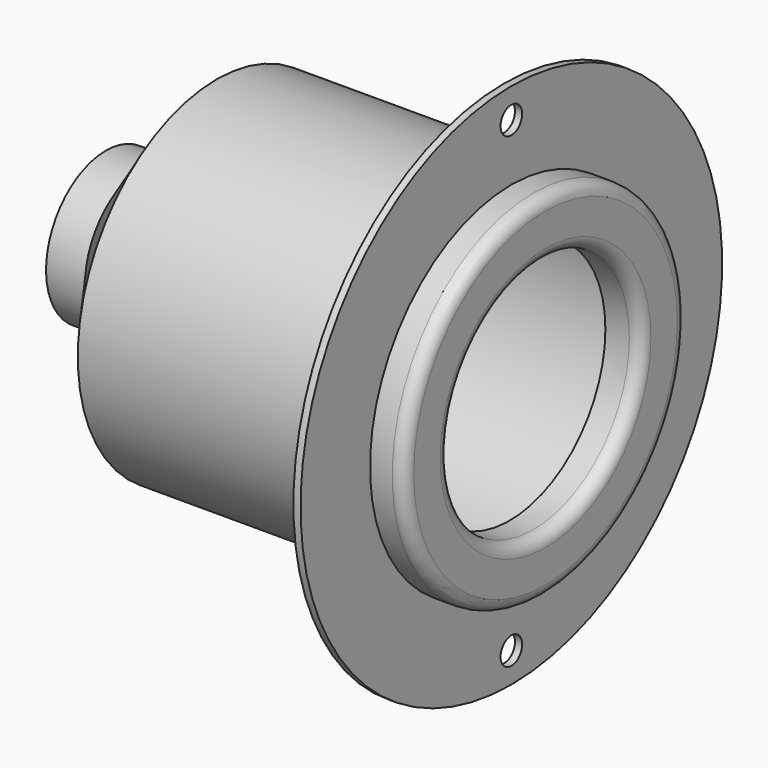
from build123d import *

# Parameters (mm, degrees)
F2_R     = 20
F3_DEPTH = 6
F4_T     = 1
F5_R     = 2
F7_D     = 4.5


# Not quite as in the source:
# - a shell that OpenCascade refuses in one call is made with other operations: the cavity is built on its own and cut out


with BuildPart() as f1:
    # F0 (on Front) → F1 (revolve)
    with BuildSketch(Plane.XZ):
        Polygon((0, 12.5), (0, 0), (73.4, 0), (73.4, 29.5), (67.7, 29.5), (67.7, 44), (66.5, 44), (66.5, 29), (18.5, 29), (6.5, 12.5), align=None)
    revolve(axis=Axis((36.7, 0, 0), (-1, 0, 0)))

    # F2 (on face) → F3 (cut)
    with BuildSketch(Plane.YZ.offset(73.4)):
        Circle(F2_R)
    extrude(amount=-F3_DEPTH, mode=Mode.SUBTRACT)

    # F4: shell of thickness 1, made by hand


with BuildPart() as f4_core1:
    # F4_t2: copy of F1
    add(f1.part)

    # the walls: a layer under each face that stays
    f4_faces = [f4_core1.faces().sort_by_distance(p)[0] for p in [
        (3.25, 0, -12.5),
        (12.5, 0, -20.75),
        (42.5, 0, -29),
        (66.5, -29.3333333333, -29.3333333333),
        (67.1, 0, -44),
        (67.7, -29.3333333333, 29.3333333333),
        (70.55, 0, -29.5),
        (73.4, -19.6666666667, 19.6666666667),
        (70.4, -20, 0),
    ]]
    thicken(f4_faces, amount=-F4_T, mode=Mode.SUBTRACT)

    # F4_s3 → F4_t4 (revolve, cut)
    with BuildSketch(Plane.XZ):
        Polygon((6.4919126392, 12.515881717), (6.5, 11.5), (7.0092245917, 11.5), (7.3087360843, 11.9118283023), align=None)
    revolve(axis=Axis((6.5, 0, 0), (-1, 0, 0)), mode=Mode.SUBTRACT)

    # F4_s5 → F4_t6 (revolve, cut)
    with BuildSketch(Plane.XZ):
        Polygon((66.49, 29.01), (66.5, 28), (67.5, 28), (67.5, 29), align=None)
    revolve(axis=Axis((66.5, 0, 0), (-1, 0, 0)), mode=Mode.SUBTRACT)

    # F4_s7 → F4_t8 (revolve, cut)
    with BuildSketch(Plane.XZ):
        Polygon((67.71, 29.51), (66.7, 29.5), (66.7, 28.5), (67.7, 28.5), align=None)
    revolve(axis=Axis((67.7, 0, 0), (-1, 0, 0)), mode=Mode.SUBTRACT)


with BuildPart() as f1_1:
    add(f1.part)

    # what is left inside the walls is the cavity
    f4_cavity = [f4_core1.part.solids().sort_by_distance(p)[0] for p in [
        (50.669742, 0, -27.99),
    ]]
    add(f4_cavity, mode=Mode.SUBTRACT)

    # F5
    f5_edges = [f1_1.edges().sort_by_distance(p)[0] for p in [
        (73.4, 0, -29.5),
        (73.4, -20, 0),
    ]]
    fillet(f5_edges, radius=F5_R)

    # F7 (through all)
    with Locations(Plane.YZ.offset(67.7)):
        with Locations((0, 39), (0, -39)):
            Hole(F7_D / 2)


solid = f1_1.part
